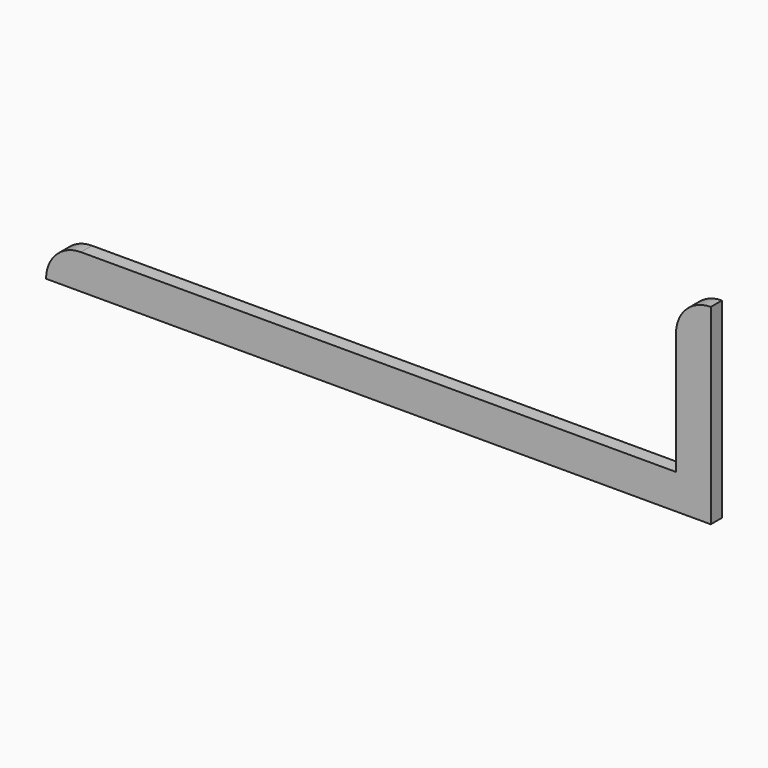
from build123d import *

# Parameters (mm, degrees)
F0_W     = 1910
F0_H     = 40
F1_DEPTH = 100
F2_W     = 100
F2_H     = 40
F3_DEPTH = 450
F4_R     = 99.99999


# Not quite as in the source:
# - a fillet or chamfer is up to 0.001 mm smaller than in the source, because OpenCascade refuses the exact size


with BuildPart() as f1:
    # F0 (on Top) → F1 (new body)
    with BuildSketch(Plane.XY):
        with Locations((10.5278193951, -112.9367578724)):
            Rectangle(F0_W, F0_H)
    extrude(amount=F1_DEPTH)

    # F2 (on face) → F3 (join)
    with BuildSketch(Plane.XY.offset(100)):
        with Locations((915.5278193951, -112.9367578724)):
            Rectangle(F2_W, F2_H)
    extrude(amount=F3_DEPTH)

    # F4 (radius 100 in the source; OpenCascade refuses exactly that, so slightly less here)
    f4_edges = [f1.edges().sort_by_distance(p)[0] for p in [
        (-944.472181, -112.936758, 100),
        (865.527819, -112.936758, 550),
    ]]
    fillet(f4_edges, radius=F4_R)


solid = f1.part
